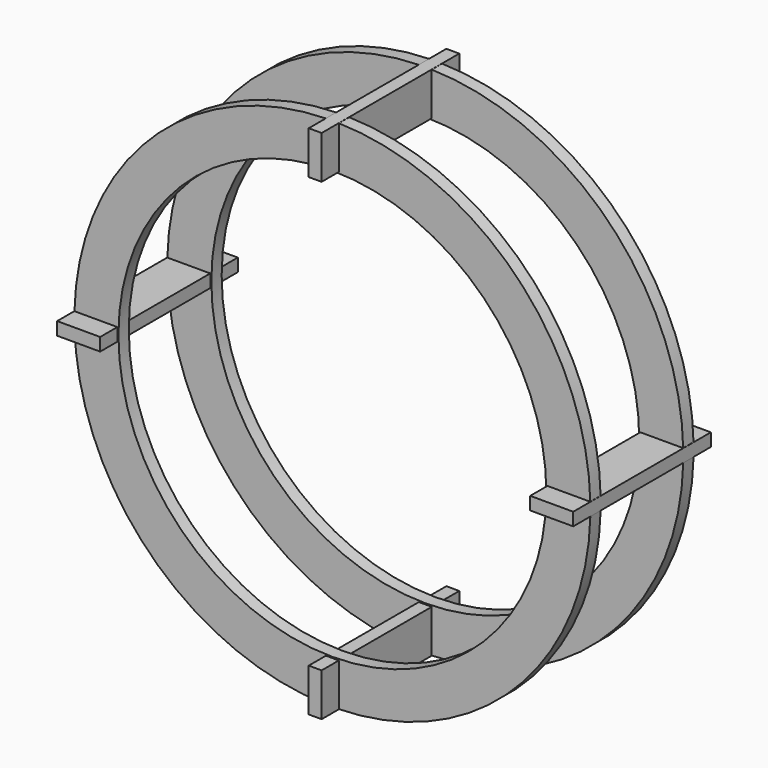
from build123d import *

# Parameters (mm, degrees)
F0_R          = 60
F0_R_2        = 49.75
F4_DEPTH      = 3
F2_R          = 60
F2_R_2        = 49.75
F5_DEPTH      = 3
F3_W          = 40
F3_H          = 10
F6_DEPTH      = 1.5
F6_DEPTH_BACK = 1.5
F7_W          = 2.6
F7_H          = 7
F7_W_2        = 7
F7_H_2        = 2.6
F8_DEPTH      = 30
F9_W          = 2.6
F9_H          = 7
F10_DEPTH     = 3
F11_COUNT     = 4


# Not quite as in the source:
# - a feature names something its author has since deleted; it is built from what else it names


with BuildPart() as f4:
    # F0 (on Front) → F4 (new body)
    with BuildSketch(Plane.XZ):
        Circle(F0_R)
        Circle(F0_R_2, mode=Mode.SUBTRACT)
    extrude(amount=F4_DEPTH)


with BuildPart() as f5:
    # F2 (on offset) → F5 (new body)
    with BuildSketch(Plane.XZ.offset(30)):
        Circle(F2_R)
        Circle(F2_R_2, mode=Mode.SUBTRACT)
    extrude(amount=-F5_DEPTH)


with BuildPart() as f6:
    # F3 (on Right) → F6 (new body, two sides)
    with BuildSketch(Plane.YZ) as f6_sk:
        with Locations((-15, 55)):
            Rectangle(F3_W, F3_H)
    extrude(amount=F6_DEPTH)
    extrude(f6_sk.sketch, amount=-F6_DEPTH_BACK)

    # F9 (on face) → F10 (cut)
    with BuildSketch(Plane.YZ.offset(1.5)):
        with Locations((-1.5, 51.5)):
            Rectangle(F9_W, F9_H)
        with Locations((-28.5, 51.5)):
            Rectangle(F9_W, F9_H)
    extrude(amount=-F10_DEPTH, mode=Mode.SUBTRACT)


with BuildPart() as f8_tool:
    # F7 (on Front) → F8 (new body)
    with BuildSketch(Plane.XZ):
        with Locations((0, 58.3)):
            Rectangle(F7_W, F7_H)
        with Locations((-58.5, 0)):
            Rectangle(F7_W_2, F7_H_2)
        with Locations((-0.2, -58.5)):
            Rectangle(F7_W, F7_H)
        with Locations((58.3, -0.2)):
            Rectangle(F7_W_2, F7_H_2)
    extrude(amount=F8_DEPTH)


with BuildPart() as f4_1:
    add(f4.part)

    # F8: cut by f8_tool
    add(f8_tool.part, mode=Mode.SUBTRACT)


with BuildPart() as f5_1:
    add(f5.part)

    # F8: cut by f8_tool
    add(f8_tool.part, mode=Mode.SUBTRACT)


with BuildPart() as f11_1:
    # F11: instance of F6
    add(f6.part.rotate(Axis((0, -30, 0), (0, -1, 0)), 1 * 360 / F11_COUNT))


with BuildPart() as f11_2:
    # F11: instance of F6
    add(f6.part.rotate(Axis((0, -30, 0), (0, -1, 0)), 2 * 360 / F11_COUNT))


with BuildPart() as f11_3:
    # F11: instance of F6
    add(f6.part.rotate(Axis((0, -30, 0), (0, -1, 0)), 3 * 360 / F11_COUNT))


solid = Compound([f6.part, f4_1.part, f5_1.part, f11_1.part, f11_2.part, f11_3.part])
